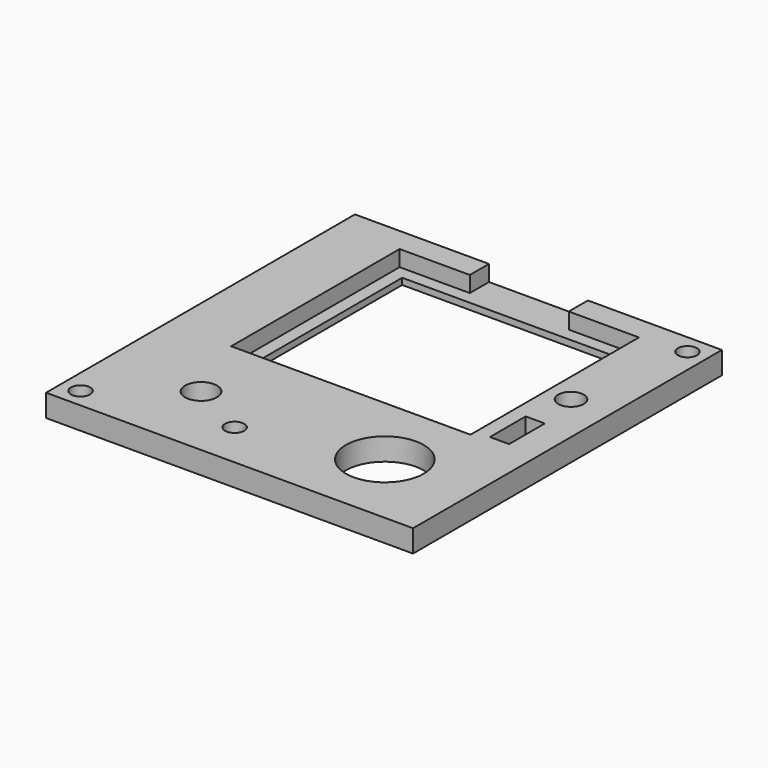
from build123d import *

# Parameters (mm, degrees)
F0_W     = 57.5
F0_H     = 60.5
F0_R     = 1.5
F0_R_2   = 2.5
F0_R_3   = 6.1
F0_W_2   = 3
F0_H_2   = 7
F0_W_3   = 37.5
F0_H_3   = 33
F0_R_4   = 2
F1_DEPTH = 3.5
F3_W     = 37.5
F3_H     = 33
F3_W_2   = 33.5
F3_H_2   = 29
F4_DEPTH = 1
F2_W     = 15.5
F2_H     = 3.75
F5_DEPTH = 2.5


with BuildPart() as f1:
    # F0 (on Top) → F1 (new body)
    with BuildSketch(Plane.XY):
        with Locations((94.6610440163, 0)):
            Rectangle(F0_W, F0_H)
        with Locations((68.9110440163, -27.25)):
            Circle(F0_R, mode=Mode.SUBTRACT)
        with Locations((89.6610440163, -23)):
            Circle(F0_R, mode=Mode.SUBTRACT)
        with Locations((80.5132240057, -18.15)):
            Circle(F0_R_2, mode=Mode.SUBTRACT)
        with Locations((109.3110440163, -18.15)):
            Circle(F0_R_3, mode=Mode.SUBTRACT)
        with Locations((117.1610440163, -2)):
            Rectangle(F0_W_2, F0_H_2, mode=Mode.SUBTRACT)
        with Locations((94.6610440163, 10)):
            Rectangle(F0_W_3, F0_H_3, mode=Mode.SUBTRACT)
        with Locations((117.1610440163, 8.5)):
            Circle(F0_R_4, mode=Mode.SUBTRACT)
        with Locations((120.4110440163, 27.25)):
            Circle(F0_R, mode=Mode.SUBTRACT)
    extrude(amount=F1_DEPTH)

    # F3 (on face) → F4 (join)
    with BuildSketch(Plane(origin=(0, 0, 0), x_dir=(1, 0, 0), z_dir=(0, 0, -1))):
        with Locations((94.6610440163, -10)):
            Rectangle(F3_W, F3_H)
        with Locations((94.6610440163, -10)):
            Rectangle(F3_W_2, F3_H_2, mode=Mode.SUBTRACT)
    extrude(amount=-F4_DEPTH)

    # F2 (on face) → F5 (cut)
    with BuildSketch(Plane.XY.offset(3.5)):
        with Locations((94.6610440163, 28.375)):
            Rectangle(F2_W, F2_H)
    extrude(amount=-F5_DEPTH, mode=Mode.SUBTRACT)


solid = f1.part
